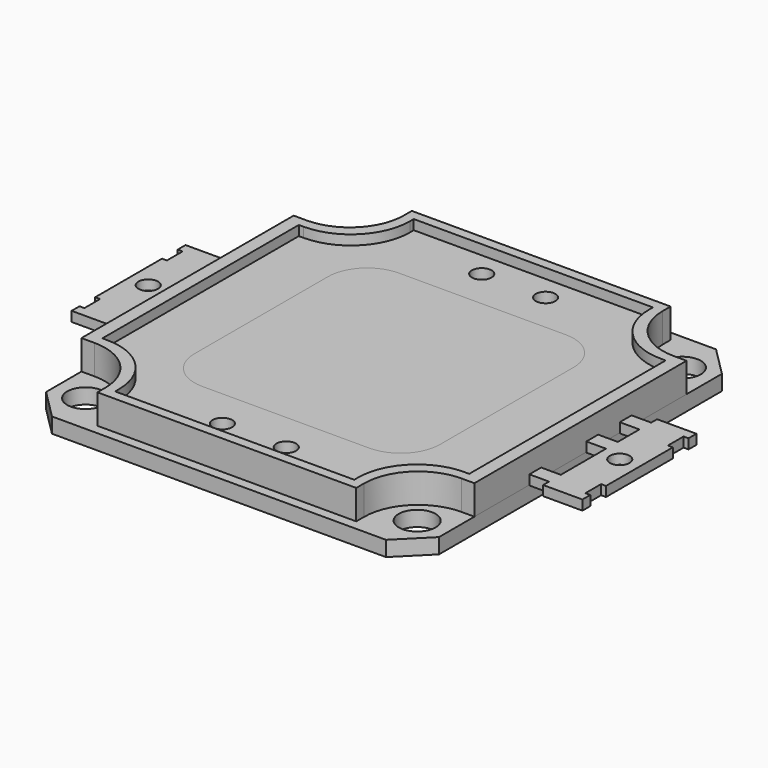
from build123d import *

# Parameters (mm, degrees)
F1_DEPTH = 1.55
F3_SIZE  = 3
F4_R     = 1.875
F5_DEPTH = 4
F6_DEPTH = 3
F2_R     = 1
F2_W     = 1.5
F2_H     = 0.5
F2_W_2   = 0.5
F2_H_2   = 1.5219762474
F2_H_3   = 1.4780237526
F7_DEPTH = 2
F8_DEPTH = 2
F9_START = 1.5
F0_W     = 2
F0_H     = 1.5
F0_R     = 1
F9_DEPTH = 1


with BuildPart() as f1:
    # F0 (on Top) → F1 (new body)
    with BuildSketch(Plane.XY):
        Polygon((20, 21), (-20, 21), (-20, 6.5), (-20, 5), (-20, 2.25), (-20, 0.75), (-20, -5), (-20, -6.5), (-20, -21), (20, -21), (20, -6.5), (20, -5), (20, 0.75), (20, 2.25), (20, 5), (20, 6.5), align=None)
    extrude(amount=F1_DEPTH)

    # F3
    f3_edges = [f1.edges().sort_by_distance(p)[0] for p in [
        (-20, 21, 0.775),
        (20, 21, 0.775),
        (20, -21, 0.775),
        (-20, -21, 0.775),
    ]]
    chamfer(f3_edges, length=F3_SIZE)

    # F4 (on face) → F5 (cut)
    with BuildSketch(Plane.XY.offset(1.55)):
        with Locations((-16.875, -16.875)):
            Circle(F4_R)
        with Locations((16.875, -16.875)):
            Circle(F4_R)
        with Locations((16.875, 16.875)):
            Circle(F4_R)
        with Locations((-16.875, 16.875)):
            Circle(F4_R)
    extrude(amount=-F5_DEPTH, mode=Mode.SUBTRACT)

    # F0 (on Top) → F9 (join)
    with BuildSketch(Plane.XY.offset(F9_START)):
        with Locations((21, 5.75)):
            Rectangle(F0_W, F0_H)
        with Locations((21, 1.5)):
            Rectangle(F0_W, F0_H)
        with Locations((-21, 5.75)):
            Rectangle(F0_W, F0_H)
        with Locations((-21, 1.5)):
            Rectangle(F0_W, F0_H)
        with Locations((-21, -5.75)):
            Rectangle(F0_W, F0_H)
        Polygon((-22, 5), (-22, 6.5), (-22, 7.25), (-26, 7.25), (-26, 6.25), (-25.5, 6.25), (-25.5, 4.25), (-26, 4.25), (-26, -4.25), (-25.5, -4.25), (-25.5, -6.25), (-26, -6.25), (-26, -7.25), (-22, -7.25), (-22, -6.5), (-22, -5), (-22, 0.75), (-22, 2.25), align=None)
        with Locations((-24, 0)):
            Circle(F0_R, mode=Mode.SUBTRACT)
        with Locations((21, -5.75)):
            Rectangle(F0_W, F0_H)
        Polygon((22, 7.25), (22, 6.5), (22, 5), (22, 2.25), (22, 0.75), (22, -5), (22, -6.5), (22, -7.25), (26, -7.25), (26, -6.25), (25.5, -6.25), (25.5, -4.25), (26, -4.25), (26, 4.25), (25.5, 4.25), (25.5, 6.25), (26, 6.25), (26, 7.25), align=None)
        with Locations((24, 0)):
            Circle(F0_R, mode=Mode.SUBTRACT)
    extrude(amount=F9_DEPTH)


with BuildPart() as f6:
    # F2 (on face) → F6 (new body)
    with BuildSketch(Plane.XY.offset(1.55)):
        with BuildLine():
            Line((13.1731458455, 20), (-13.1731458455, 20))
            Line((-13.1731458455, 20), (-13.1731458455, 19))
            ThreePointArc((-13.1731458455, 19), (-14.784058549, 15.1109127035), (-18.6731458455, 13.5))
            Line((-18.6731458455, 13.5), (-20, 13.5))
            Line((-20, 13.5), (-20, -13.5))
            Line((-20, -13.5), (-18.6731458455, -13.5))
            ThreePointArc((-18.6731458455, -13.5), (-14.784058549, -15.1109127035), (-13.1731458455, -19))
            Line((-13.1731458455, -19), (-13.1731458455, -20))
            Line((-13.1731458455, -20), (13.1731458455, -20))
            Line((13.1731458455, -20), (13.1731458455, -19))
            ThreePointArc((13.1731458455, -19), (14.784058549, -15.1109127035), (18.6731458455, -13.5))
            Line((18.6731458455, -13.5), (20, -13.5))
            Line((20, -13.5), (20, 13.5))
            Line((20, 13.5), (18.6731458455, 13.5))
            ThreePointArc((18.6731458455, 13.5), (14.784058549, 15.1109127035), (13.1731458455, 19))
            Line((13.1731458455, 19), (13.1731458455, 20))
        make_face()
        with BuildLine():
            Line((-12.1731458455, 18.5), (-12.1731458455, 19))
            Line((-12.1731458455, 19), (12.1731458455, 19))
            Line((12.1731458455, 19), (12.1731458455, 18.5))
            ThreePointArc((12.1731458455, 18.5), (13.9305051584, 14.2573593129), (18.1731458455, 12.5))
            Line((18.1731458455, 12.5), (18.6731458455, 12.5))
            Line((18.6731458455, 12.5), (18.6731458455, -12.5))
            Line((18.6731458455, -12.5), (18.1731458455, -12.5))
            ThreePointArc((18.1731458455, -12.5), (13.9305051584, -14.2573593129), (12.1731458455, -18.5))
            Line((12.1731458455, -18.5), (12.1731458455, -19))
            Line((12.1731458455, -19), (-12.1731458455, -19))
            Line((-12.1731458455, -19), (-12.1731458455, -18.5))
            ThreePointArc((-12.1731458455, -18.5), (-13.9305051584, -14.2573593129), (-18.1731458455, -12.5))
            Line((-18.1731458455, -12.5), (-18.6731458455, -12.5))
            Line((-18.6731458455, -12.5), (-18.6731458455, 12.5))
            Line((-18.6731458455, 12.5), (-18.1731458455, 12.5))
            ThreePointArc((-18.1731458455, 12.5), (-13.9305051584, 14.2573593129), (-12.1731458455, 18.5))
        make_face(mode=Mode.SUBTRACT)
    extrude(amount=F6_DEPTH)

    # F2 (on face) → F7 (join)
    with BuildSketch(Plane.XY.offset(1.55)):
        with BuildLine():
            Line((12.1731458455, 19), (-12.1731458455, 19))
            Line((-12.1731458455, 19), (-12.1731458455, 18.5))
            ThreePointArc((-12.1731458455, 18.5), (-13.9305051584, 14.2573593129), (-18.1731458455, 12.5))
            Line((-18.1731458455, 12.5), (-18.6731458455, 12.5))
            Line((-18.6731458455, 12.5), (-18.6731458455, -12.5))
            Line((-18.6731458455, -12.5), (-18.1731458455, -12.5))
            ThreePointArc((-18.1731458455, -12.5), (-13.9305051584, -14.2573593129), (-12.1731458455, -18.5))
            Line((-12.1731458455, -18.5), (-12.1731458455, -19))
            Line((-12.1731458455, -19), (12.1731458455, -19))
            Line((12.1731458455, -19), (12.1731458455, -18.5))
            ThreePointArc((12.1731458455, -18.5), (13.9305051584, -14.2573593129), (18.1731458455, -12.5))
            Line((18.1731458455, -12.5), (18.6731458455, -12.5))
            Line((18.6731458455, -12.5), (18.6731458455, 12.5))
            Line((18.6731458455, 12.5), (18.1731458455, 12.5))
            ThreePointArc((18.1731458455, 12.5), (13.9305051584, 14.2573593129), (12.1731458455, 18.5))
            Line((12.1731458455, 18.5), (12.1731458455, 19))
        make_face()
        Polygon((-9.1731458455, -16.4780237526), (-9.1731458455, -18), (-9.6731458455, -18), (-9.6731458455, -16.4780237526), (-11.1731458455, -16.4780237526), (-11.1731458455, -15.9780237526), (-9.6731458455, -15.9780237526), (-9.6731458455, -14.5), (-9.1731458455, -14.5), (-9.1731458455, -15.9780237526), (-7.6731458455, -15.9780237526), (-7.6731458455, -16.4780237526), align=None, mode=Mode.SUBTRACT)
        with Locations((-3.25, -16.5)):
            Circle(F2_R, mode=Mode.SUBTRACT)
        with Locations((3.25, -16.5)):
            Circle(F2_R, mode=Mode.SUBTRACT)
        with Locations((-3.25, 16.5)):
            Circle(F2_R, mode=Mode.SUBTRACT)
        with BuildLine():
            ThreePointArc((-12.5, 8.5), (-11.3284271247, 11.3284271247), (-8.5, 12.5))
            Line((-8.5, 12.5), (8.5, 12.5))
            ThreePointArc((8.5, 12.5), (11.3284271247, 11.3284271247), (12.5, 8.5))
            Line((12.5, 8.5), (12.5, -8.5))
            ThreePointArc((12.5, -8.5), (11.3284271247, -11.3284271247), (8.5, -12.5))
            Line((8.5, -12.5), (-8.5, -12.5))
            ThreePointArc((-8.5, -12.5), (-11.3284271247, -11.3284271247), (-12.5, -8.5))
            Line((-12.5, -8.5), (-12.5, 8.5))
        make_face(mode=Mode.SUBTRACT)
        with Locations((3.25, 16.5)):
            Circle(F2_R, mode=Mode.SUBTRACT)
        with Locations((-8.4231458455, -16.2280237526)):
            Rectangle(F2_W, F2_H)
        with Locations((-10.4231458455, -16.2280237526)):
            Rectangle(F2_W, F2_H)
        with Locations((-9.4231458455, -17.2390118763)):
            Rectangle(F2_W_2, F2_H_2)
        with Locations((-9.4231458455, -15.2390118763)):
            Rectangle(F2_W_2, F2_H_3)
        with Locations((-9.4231458455, -16.2280237526)):
            Rectangle(F2_W_2, F2_H)
    extrude(amount=F7_DEPTH)


with BuildPart() as f8:
    # F2 (on face) → F8 (new body)
    with BuildSketch(Plane.XY.offset(1.55)):
        with BuildLine():
            Line((8.5, 12.5), (-8.5, 12.5))
            ThreePointArc((-8.5, 12.5), (-11.3284271247, 11.3284271247), (-12.5, 8.5))
            Line((-12.5, 8.5), (-12.5, -8.5))
            ThreePointArc((-12.5, -8.5), (-11.3284271247, -11.3284271247), (-8.5, -12.5))
            Line((-8.5, -12.5), (8.5, -12.5))
            ThreePointArc((8.5, -12.5), (11.3284271247, -11.3284271247), (12.5, -8.5))
            Line((12.5, -8.5), (12.5, 8.5))
            ThreePointArc((12.5, 8.5), (11.3284271247, 11.3284271247), (8.5, 12.5))
        make_face()
    extrude(amount=F8_DEPTH)


solid = Compound([f1.part, f6.part, f8.part])
